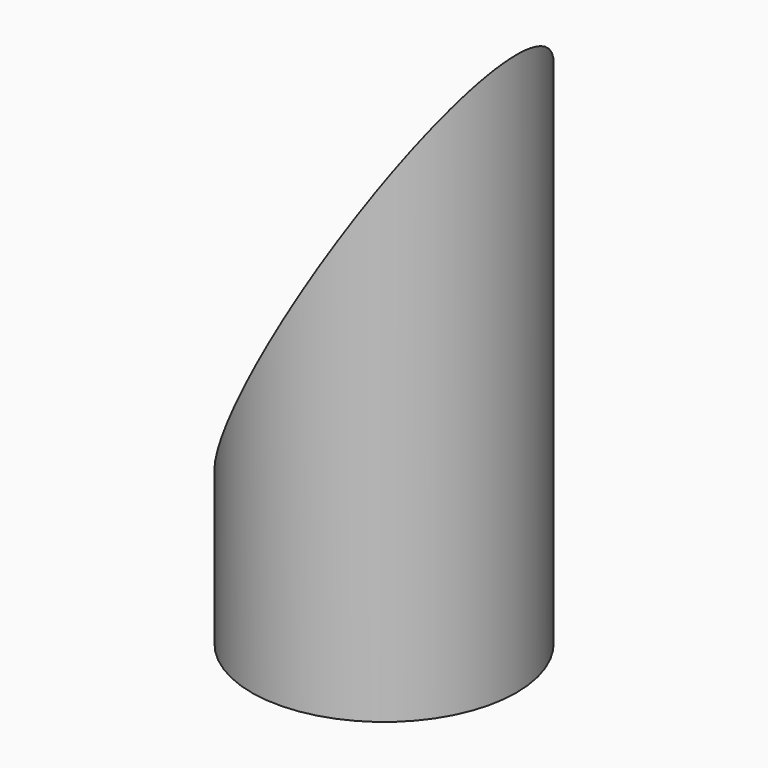
from build123d import *

# Parameters (mm, degrees)
F0_R         = 19.05
F0_R_2       = 12.7635
F1_DEPTH     = 88.9
F3_DEPTH     = 63.5
F4_TEXT_SIZE = 5.6430448797
F5_DEPTH     = 2.54


# Not quite as in the source:
# - Text() gives the source's letters only with a copy of the font that has no kerning and outlines rounded to 1/6400 em; it was checked with that copy


with BuildPart() as f1:
    # F0 (on Top) → F1 (new body)
    with BuildSketch(Plane.XY):
        Circle(F0_R)
        Circle(F0_R_2, mode=Mode.SUBTRACT)
    extrude(amount=F1_DEPTH)

    # F2 (on Front) → F3 (cut, symmetric)
    with BuildSketch(Plane.XZ):
        Polygon((-29.6211251989, -3.5522840917), (35.9570560977, 110.0324577819), (-33.1656448543, 110.0324577819), align=None)
    extrude(amount=F3_DEPTH, both=True, mode=Mode.SUBTRACT)

    # F4 (on face) → F5 (cut)
    with BuildSketch(Plane(origin=(-20.6776597667, 0, 11.9382524325), x_dir=(0, -1, 0), z_dir=(-0.8660254038, 0, 0.5))):
        with Locations((-8.89, 9.3565442511)):
            Text('30DEG', F4_TEXT_SIZE, font='Open Sans', font_style=FontStyle.BOLD, text_align=(TextAlign.LEFT, TextAlign.BOTTOM))
    extrude(amount=-F5_DEPTH, mode=Mode.SUBTRACT)


solid = f1.part
